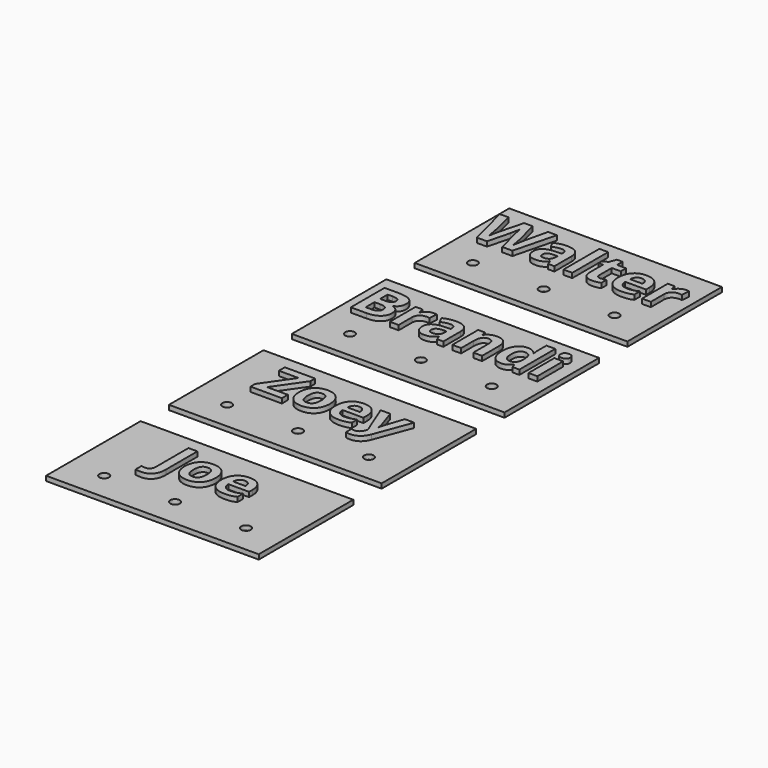
from build123d import *

# Parameters (mm, degrees)
F0_W         = 90
F0_H         = 50
F0_R         = 2
F1_DEPTH     = 2
F2_TEXT_SIZE = 25
F3_DEPTH     = 2
F4_TEXT_SIZE = 25
F5_DEPTH     = 2
F6_TEXT_SIZE = 25
F7_DEPTH     = 2
F8_TEXT_SIZE = 25
F9_DEPTH     = 2


# Not quite as in the source:
# - Text() gives the source's letters only with a copy of the font that has no kerning and outlines rounded to 1/6400 em; it was checked with that copy


with BuildPart() as f1:
    # F0 (on Top) → F1 (new body)
    with BuildSketch(Plane.XY):
        with Locations((-4.1558017731, 20.6805696711)):
            Rectangle(F0_W, F0_H)
        with Locations((-34.1558017731, 7.6805696711)):
            Circle(F0_R, mode=Mode.SUBTRACT)
        with Locations((-4.1558017731, 7.6805696711)):
            Circle(F0_R, mode=Mode.SUBTRACT)
        with Locations((25.8441982269, 7.6805696711)):
            Circle(F0_R, mode=Mode.SUBTRACT)
    extrude(amount=-F1_DEPTH)

    # F2 (on face) → F3 (join)
    with BuildSketch(Plane.XY):
        with Locations((-46.6421298981, 19.6805696711)):
            Text('Walter', F2_TEXT_SIZE, font='Open Sans', font_style=FontStyle.BOLD, text_align=(TextAlign.LEFT, TextAlign.BOTTOM))
    extrude(amount=F3_DEPTH)


with BuildPart() as f1b:
    # F0 (on Top) → F1, piece 2 (new body)
    with BuildSketch(Plane.XY):
        with Locations((-4.1558017731, -44.3194303289)):
            Rectangle(F0_W, F0_H)
        with Locations((-34.1558017731, -57.3194303289)):
            Circle(F0_R, mode=Mode.SUBTRACT)
        with Locations((-4.1558017731, -57.3194303289)):
            Circle(F0_R, mode=Mode.SUBTRACT)
        with Locations((25.8441982269, -57.3194303289)):
            Circle(F0_R, mode=Mode.SUBTRACT)
    extrude(amount=-F1_DEPTH)

    # F4 (on face) → F5 (join)
    with BuildSketch(Plane.XY):
        with Locations((-45.6401767731, -45.3194303289)):
            Text('Brandi', F4_TEXT_SIZE, font='Open Sans', font_style=FontStyle.BOLD, text_align=(TextAlign.LEFT, TextAlign.BOTTOM))
    extrude(amount=F5_DEPTH)


with BuildPart() as f1c:
    # F0 (on Top) → F1, piece 3 (new body)
    with BuildSketch(Plane.XY):
        with Locations((-4.1558017731, -109.3194303289)):
            Rectangle(F0_W, F0_H)
        with Locations((-34.1558017731, -122.3194303289)):
            Circle(F0_R, mode=Mode.SUBTRACT)
        with Locations((-4.1558017731, -122.3194303289)):
            Circle(F0_R, mode=Mode.SUBTRACT)
        with Locations((25.8441982269, -122.3194303289)):
            Circle(F0_R, mode=Mode.SUBTRACT)
    extrude(amount=-F1_DEPTH)

    # F6 (on face) → F7 (join)
    with BuildSketch(Plane.XY):
        with Locations((-34.4409580231, -110.3194303289)):
            Text('Zoey', F6_TEXT_SIZE, font='Open Sans', font_style=FontStyle.BOLD, text_align=(TextAlign.LEFT, TextAlign.BOTTOM))
    extrude(amount=F7_DEPTH)


with BuildPart() as f1d:
    # F0 (on Top) → F1, piece 4 (new body)
    with BuildSketch(Plane.XY):
        with Locations((-4.1558017731, -174.3194303289)):
            Rectangle(F0_W, F0_H)
        with Locations((-34.1558017731, -187.3194303289)):
            Circle(F0_R, mode=Mode.SUBTRACT)
        with Locations((-4.1558017731, -187.3194303289)):
            Circle(F0_R, mode=Mode.SUBTRACT)
        with Locations((25.8441982269, -187.3194303289)):
            Circle(F0_R, mode=Mode.SUBTRACT)
    extrude(amount=-F1_DEPTH)

    # F8 (on face) → F9 (join)
    with BuildSketch(Plane.XY):
        with Locations((-24.6206455231, -175.3194303289)):
            Text('Joe', F8_TEXT_SIZE, font='Open Sans', font_style=FontStyle.BOLD, text_align=(TextAlign.LEFT, TextAlign.BOTTOM))
    extrude(amount=F9_DEPTH)


solid = Compound([f1.part, f1b.part, f1c.part, f1d.part])
